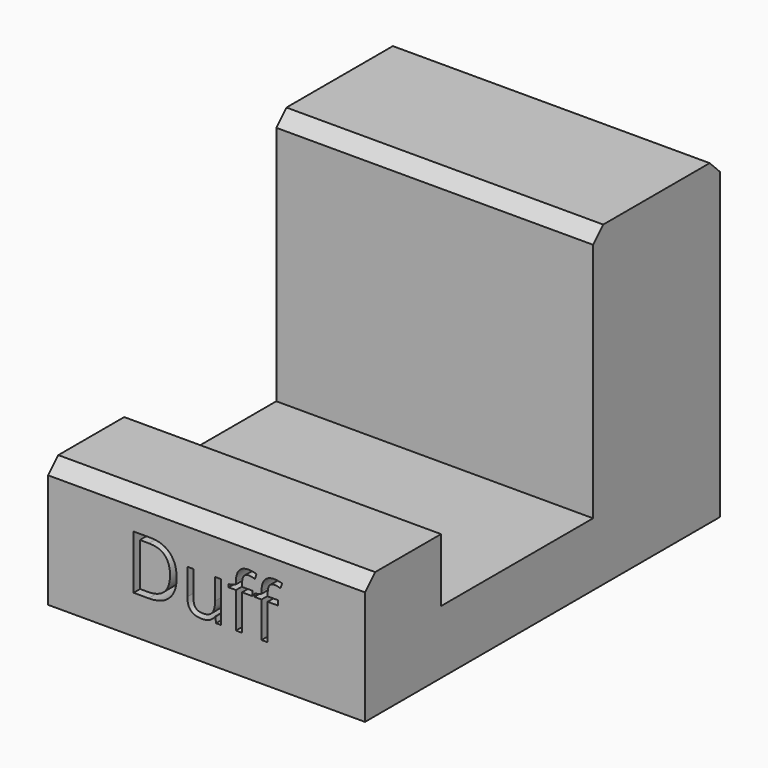
from build123d import *

# Parameters (mm, degrees)
F1_DEPTH     = 25
F2_TEXT_SIZE = 11.9243438045
F3_DEPTH     = 10
F4_SIZE      = 2


# Not quite as in the source:
# - Text() gives the source's letters only with a copy of the font that has no kerning and outlines rounded to 1/6400 em; it was checked with that copy


with BuildPart() as f1:
    # F0 (on Right) → F1 (new body, symmetric)
    with BuildSketch(Plane.YZ):
        Polygon((-25.4561832547, 20), (-40.4561832547, 20), (-40.4561832547, 0), (29.5438167453, 0), (29.5438167453, 50), (4.5438167453, 50), (4.5438167453, 10), (-25.4561832547, 10), align=None)
    extrude(amount=F1_DEPTH, both=True)

    # F2 (on face) → F3 (cut)
    with BuildSketch(Plane.XZ.offset(40.4561832547)):
        with Locations((-12.6901102582, 6.0690790415)):
            Text('Duff', F2_TEXT_SIZE, font='Open Sans', text_align=(TextAlign.LEFT, TextAlign.BOTTOM))
    extrude(amount=-F3_DEPTH, mode=Mode.SUBTRACT)

    # F4
    f4_edges = [f1.edges().sort_by_distance(p)[0] for p in [
        (0, -40.456183, 20),
        (0, 29.543817, 50),
        (0, 4.543817, 50),
    ]]
    chamfer(f4_edges, length=F4_SIZE)


solid = f1.part
